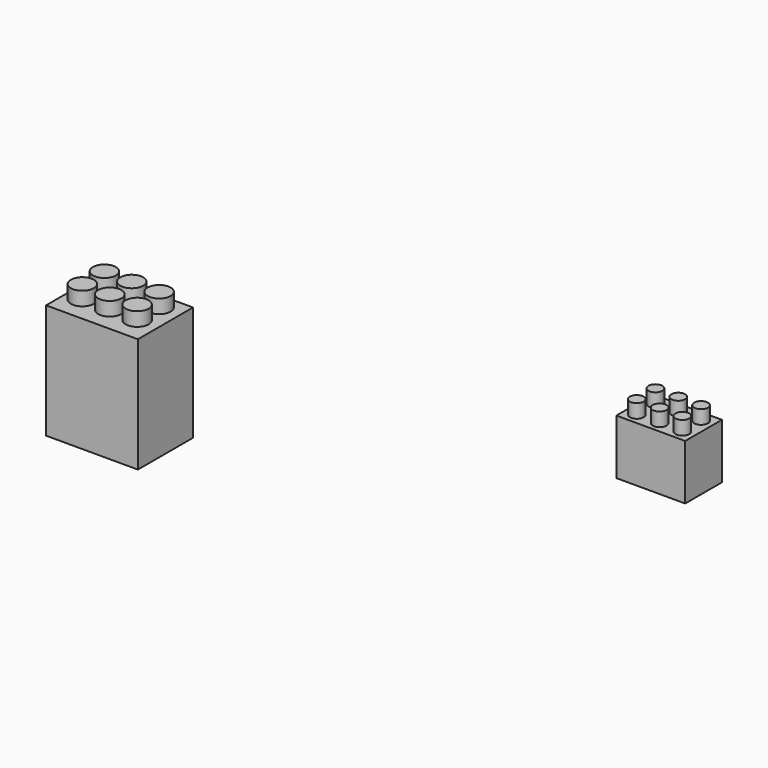
from build123d import *

# Parameters (mm, degrees)
F0_W     = 15
F0_H     = 10
F1_DEPTH = 12
F2_R     = 1.5
F3_DEPTH = 3
F4_W     = 20
F4_H     = 15
F5_DEPTH = 25
F6_R     = 2.5
F7_DEPTH = 3
F8_W     = 14.1492537223
F8_H     = 9.1035095975
F9_DEPTH = 8


# Not quite as in the source:
# - the program builds the solid bodies; features that only make, move or delete a surface that nothing else refers to are left out


with BuildPart() as f1:
    # F0 (on Top) → F1 (new body)
    with BuildSketch(Plane.XY):
        Rectangle(F0_W, F0_H)
    extrude(amount=F1_DEPTH)

    # F2 (on face) → F3 (join)
    with BuildSketch(Plane.XY.offset(12)):
        with Locations((-4.9661255717, -2.5968982129)):
            Circle(F2_R)
        with Locations((-4.9661255717, 2.4878393313)):
            Circle(F2_R)
        with Locations((0, 2.4878393313)):
            Circle(F2_R)
        with Locations((0, -2.5968982129)):
            Circle(F2_R)
        with Locations((4.9661255717, -2.5968982129)):
            Circle(F2_R)
        with Locations((4.9661255717, 2.4878393313)):
            Circle(F2_R)
    extrude(amount=F3_DEPTH)

    # F8 (on face) → F9 (cut)
    with BuildSketch(Plane(origin=(0, 0, 0), x_dir=(1, 0, 0), z_dir=(0, 0, -1))):
        with Locations((-0.0008016359, 0.0008624047)):
            Rectangle(F8_W, F8_H)
    extrude(amount=-F9_DEPTH, mode=Mode.SUBTRACT)


with BuildPart() as f5:
    # F4 (on Top) → F5 (new body)
    with BuildSketch(Plane.XY):
        with Locations((-83.0038021637, -45.8922367543)):
            Rectangle(F4_W, F4_H)
    extrude(amount=F5_DEPTH)

    # F6 (on face) → F7 (join)
    with BuildSketch(Plane.XY.offset(25)):
        with Locations((-89.5038021637, -47.8922367543)):
            Circle(F6_R)
        with Locations((-89.5038021637, -41.8922367543)):
            Circle(F6_R)
        with Locations((-83.5039313242, -47.9316056411)):
            Circle(F6_R)
        with Locations((-83.5039313242, -41.9316056411)):
            Circle(F6_R)
        with Locations((-77.5040604847, -47.9709745279)):
            Circle(F6_R)
        with Locations((-77.5040604847, -41.9709745279)):
            Circle(F6_R)
    extrude(amount=F7_DEPTH)


solid = Compound([f1.part, f5.part])
